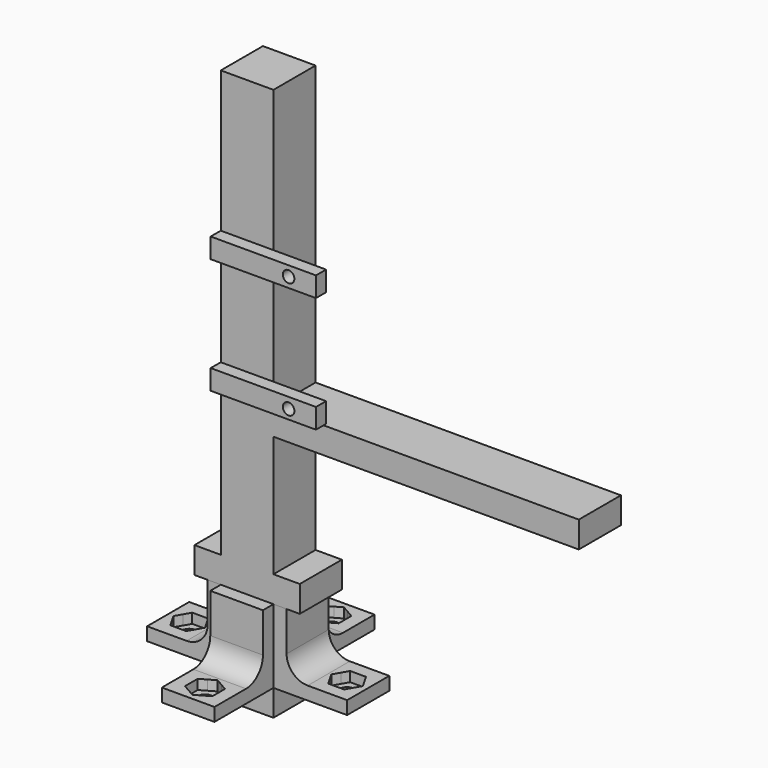
from build123d import *

# Parameters (mm, degrees)
F0_W      = 12.7
F0_H      = 12.7
F1_DEPTH  = 127
F3_DEPTH  = 12.7
F5_DEPTH  = 2.38125
F6_DEPTH  = 25.4
F8_COUNT  = 4
F9_DEPTH  = 6.35
F10_W     = 73.66
F10_H     = 6.35
F11_DEPTH = 12.7
F12_W     = 6.35
F12_H     = 6.35
F13_DEPTH = 12.7
F15_DEPTH = 3.048


# Not quite as in the source:
# - a length typed as a fraction of an inch, garbled in the dataset ("3 / 203.2 mm" for 3/8 in), is restored


with BuildPart() as f1:
    # F0 (on Top) → F1 (new body)
    with BuildSketch(Plane.XY):
        Rectangle(F0_W, F0_H)
    extrude(amount=F1_DEPTH)

    # F0 (on Top) → F9 (join)
    with BuildSketch(Plane.XY):
        Rectangle(F0_W, F0_H)
    extrude(amount=-F9_DEPTH)

    # F10 (on face) → F11 (join)
    with BuildSketch(Plane.XZ.offset(6.35)):
        with Locations((43.18, 56.515)):
            Rectangle(F10_W, F10_H)
    extrude(amount=-F11_DEPTH)

    # F12 (on face) → F13 (join)
    with BuildSketch(Plane.XZ.offset(6.35)):
        with Locations((9.525, 20.955)):
            Rectangle(F12_W, F12_H)
        with Locations((-9.525, 20.955)):
            Rectangle(F12_W, F12_H)
    extrude(amount=-F13_DEPTH)

    # F14 (on face) → F15 (join)
    with BuildSketch(Plane.XZ.offset(6.35)):
        Polygon((-6.35, 60.198), (6.35, 60.198), (19.05, 60.198), (19.05, 65.024), (6.35, 65.024), (-6.35, 65.024), align=None)
        with BuildLine():
            ThreePointArc((11.049, 62.4654579298), (12.446, 63.8624579298), (13.843, 62.4654579298))
            ThreePointArc((13.843, 62.4654579298), (12.446, 61.0684579298), (11.049, 62.4654579298))
        make_face(mode=Mode.SUBTRACT)
        Polygon((-6.35, 88.138), (6.35, 88.138), (19.05, 88.138), (19.05, 92.964), (6.35, 92.964), (-6.35, 92.964), align=None)
        with BuildLine():
            ThreePointArc((11.049, 90.551), (12.446, 91.948), (13.843, 90.551))
            ThreePointArc((13.843, 90.551), (12.446, 89.154), (11.049, 90.551))
        make_face(mode=Mode.SUBTRACT)
    extrude(amount=F15_DEPTH)


with BuildPart() as f3:
    # F2 (on face) → F3 (new body)
    with BuildSketch(Plane.XZ.offset(6.35)):
        with BuildLine():
            Line((6.35, 17.78), (6.35, 0))
            Line((6.35, 0), (24.13, 0))
            Line((24.13, 0), (24.13, 3.175))
            Line((24.13, 3.175), (14.605, 3.175))
            ThreePointArc((14.605, 3.175), (11.0128975516, 4.6628975516), (9.525, 8.255))
            Line((9.525, 8.255), (9.525, 17.78))
            Line((9.525, 17.78), (6.35, 17.78))
        make_face()
    extrude(amount=-F3_DEPTH)

    # F4 (on face) → F5 (cut)
    with BuildSketch(Plane.XY.offset(3.175)):
        with BuildLine():
            Line((16.1903839544, 1.6509997189), (15.2371788223, 0))
            Line((15.2371788223, 0), (15.748, 0))
            ThreePointArc((15.748, 0), (15.8605128796, 0.8546203301), (16.1903839544, 1.6509997189))
        make_face()
        with BuildLine():
            Line((15.748, 0), (15.2371788223, 0))
            Line((15.2371788223, 0), (16.1903839566, -1.6509997228))
            ThreePointArc((16.1903839566, -1.6509997228), (15.8605128802, -0.8546203323), (15.748, 0))
        make_face()
        with BuildLine():
            ThreePointArc((16.1903839544, 1.6509997189), (15.8605128796, 0.8546203301), (15.748, 0))
            ThreePointArc((15.748, 0), (15.8605128802, -0.8546203323), (16.1903839566, -1.6509997228))
            ThreePointArc((16.1903839566, -1.6509997228), (17.3989998614, -2.8596158033), (19.05, -3.302))
            ThreePointArc((19.05, -3.302), (20.7010000158, -2.8596158742), (21.9096159015, -1.6509999684))
            ThreePointArc((21.9096159015, -1.6509999684), (22.2394870831, -0.8546204693), (22.352, 0))
            ThreePointArc((22.352, 0), (22.2394870807, 0.8546204785), (21.9096158921, 1.6509999848))
            ThreePointArc((21.9096158921, 1.6509999848), (20.7010000076, 2.8596158789), (19.05, 3.302))
            ThreePointArc((19.05, 3.302), (17.3989998594, 2.8596158021), (16.1903839544, 1.6509997189))
        make_face()
        with BuildLine():
            ThreePointArc((20.828, 0), (19.05, -1.778), (17.272, 0))
            ThreePointArc((17.272, 0), (19.05, 1.778), (20.828, 0))
        make_face(mode=Mode.SUBTRACT)
        with BuildLine():
            ThreePointArc((19.05, -3.302), (17.3989998614, -2.8596158033), (16.1903839566, -1.6509997228))
            Line((16.1903839566, -1.6509997228), (17.1435894111, -3.302))
            Line((17.1435894111, -3.302), (19.05, -3.302))
        make_face()
        with BuildLine():
            Line((17.1435894111, 3.302), (16.1903839544, 1.6509997189))
            ThreePointArc((16.1903839544, 1.6509997189), (17.3989998594, 2.8596158021), (19.05, 3.302))
            Line((19.05, 3.302), (17.1435894111, 3.302))
        make_face()
        with BuildLine():
            ThreePointArc((21.9096159015, -1.6509999684), (20.7010000158, -2.8596158742), (19.05, -3.302))
            Line((19.05, -3.302), (20.9564105889, -3.302))
            Line((20.9564105889, -3.302), (21.9096159015, -1.6509999684))
        make_face()
        with BuildLine():
            Line((20.9564105889, 3.302), (19.05, 3.302))
            ThreePointArc((19.05, 3.302), (20.7010000076, 2.8596158789), (21.9096158921, 1.6509999848))
            Line((21.9096158921, 1.6509999848), (20.9564105889, 3.302))
        make_face()
        with BuildLine():
            ThreePointArc((22.352, 0), (22.2394870831, -0.8546204693), (21.9096159015, -1.6509999684))
            Line((21.9096159015, -1.6509999684), (22.8628211777, 0))
            Line((22.8628211777, 0), (21.9096158921, 1.6509999848))
            ThreePointArc((21.9096158921, 1.6509999848), (22.2394870807, 0.8546204785), (22.352, 0))
        make_face()
    extrude(amount=-F5_DEPTH, mode=Mode.SUBTRACT)

    # F4 (on face) → F6 (cut)
    with BuildSketch(Plane.XY.offset(3.175)):
        with BuildLine():
            ThreePointArc((20.828, 0), (19.05, 1.778), (17.272, 0))
            ThreePointArc((17.272, 0), (19.05, -1.778), (20.828, 0))
        make_face()
    extrude(amount=-F6_DEPTH, mode=Mode.SUBTRACT)


with BuildPart() as f8_1:
    # F8: instance of F3
    add(f3.part.rotate(Axis((0, 0, 41.5546000004), (0, 0, -1)), 1 * 360 / F8_COUNT))


with BuildPart() as f8_2:
    # F8: instance of F3
    add(f3.part.rotate(Axis((0, 0, 41.5546000004), (0, 0, -1)), 2 * 360 / F8_COUNT))


with BuildPart() as f8_3:
    # F8: instance of F3
    add(f3.part.rotate(Axis((0, 0, 41.5546000004), (0, 0, -1)), 3 * 360 / F8_COUNT))


solid = Compound([f1.part, f3.part, f8_1.part, f8_2.part, f8_3.part])
